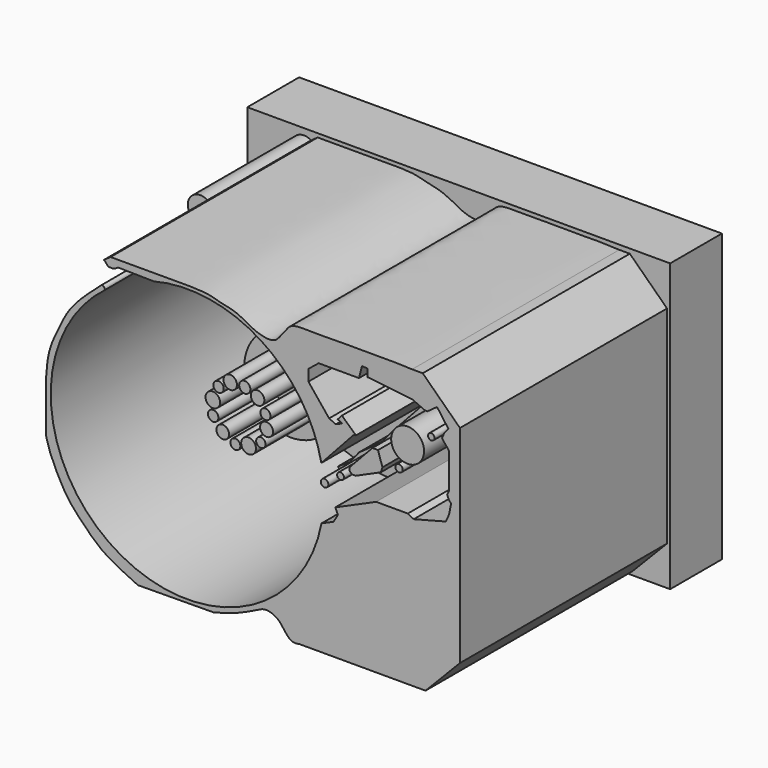
from build123d import *

# Parameters (mm, degrees)
F0_W     = 165.9392981062
F0_H     = 112.5707998872
F1_DEPTH = 25.4
F0_R     = 18.362033197
F2_DEPTH = 25.4
F0_R_2   = 1.3245760179
F0_R_3   = 1.6180887527
F0_R_4   = 1.5016288639
F0_R_5   = 1.5308685242
F0_R_6   = 1.423680284
F0_R_7   = 1.8647629935
F0_R_8   = 2.0434590637
F3_DEPTH = 101.6
F0_R_9   = 2.8584843347
F0_R_10  = 2.033776086
F0_R_11  = 2.6280999476
F0_R_12  = 2.1900875489
F0_R_13  = 2.646289047
F0_R_14  = 1.983205802
F0_R_15  = 2.5672784981
F0_R_16  = 1.8338916461
F0_R_17  = 2.9015877895
F0_R_18  = 1.9588755687
F0_R_19  = 2.4970768298
F0_R_20  = 1.4334147906
F0_R_21  = 6.4546403477
F0_R_22  = 1.275539693
F0_R_23  = 1.4866669549
F0_R_24  = 1.3335540023
F4_DEPTH = 76.2
F0_R_25  = 2.3077206763
F5_DEPTH = 127


# Not quite as in the source:
# - a feature names something its author has since deleted; it is built from what else it names


with BuildPart() as f1:
    # F0 (on Front) → F1 (new body)
    with BuildSketch(Plane.XZ):
        with Locations((-83.9341042461, -56.6721437499)):
            Rectangle(F0_W, F0_H)
        with BuildLine():
            add(Edge.make_bspline(
                [(-164.598762989, -71.9534307718), (-164.6019804727, -70.301781771), (-164.6090784651, -66.6581294606), (-164.5482157868, -58.819482394), (-164.7950691846, -52.0330130517), (-163.7374427264, -41.4198242134), (-160.0827700828, -34.2963401288), (-156.4790843754, -26.1909418494), (-150.7406910055, -19.6763424087), (-145.530215111, -15.0828061332), (-142.7876929211, -12.6653148558)],
                knots=[0, 0, 0, 0, 0.1000210606, 0.2206534006, 0.3367660722, 0.4769540157, 0.6014757189, 0.7294078454, 0.8575200865, 0.9998406243, 0.9998406243, 0.9998406243, 0.9998406243], degree=3))
            add(Edge.make_bspline(
                [(-143.3946741623, -12.5450599833), (-143.1883174895, -12.5826121553), (-142.9822493327, -12.6205904733), (-142.7876929211, -12.6653148558)],
                knots=[0, 0, 0, 0, 0.1891030532, 0.1891030532, 0.1891030532, 0.1891030532], degree=3))
            ThreePointArc((-143.3946741623, -12.5450599833), (-149.5463977213, -6.9914400334), (-141.9263395611, -3.7324354414))
            Line((-141.9263395611, -3.7324354414), (-139.2825245857, -1.8620226765))
            add(Edge.make_bspline(
                [(-139.2825245857, -1.8620226765), (-136.5395607147, -1.8628613769), (-130.4584942921, -1.8647207497), (-117.4190427855, -1.8500489741), (-110.495055532, -1.8905468427), (-106.0578439103, -1.7735924347), (-100.2520493143, -2.2187206408), (-96.5814322262, -3.5750412815), (-91.8177960869, -4.2369226936), (-87.1565766192, -6.2408038722), (-83.7146728479, -8.3917462542), (-80.2039650745, -9.7577587847), (-74.7501088384, -10.6611105909), (-72.0211091883, -6.5408088644), (-70.0817167302, -4.1727022961), (-67.8282888978, -1.5520558306), (-57.6837259787, -2.2476289823), (-49.8219729842, -1.7591343826), (-37.8466777831, -2.1896007905), (-29.9600520641, -1.7316118376), (-23.4707458973, -2.1886006133), (-20.9419615567, -2.1850855555)],
                knots=[0, 0, 0, 0, 0.0604152758, 0.1339388058, 0.1870270437, 0.2294758615, 0.2776594332, 0.3179706024, 0.3620093694, 0.4077635186, 0.4481802316, 0.4879171376, 0.5330108477, 0.5757838582, 0.6112628399, 0.6462449623, 0.7084529789, 0.7682332833, 0.8371419361, 0.8957157052, 0.9554909702, 0.9554909702, 0.9554909702, 0.9554909702], degree=3))
            Line((-20.9419615567, -2.1850855555), (-16.7830623686, -2.1850855555))
            Line((-16.7830623686, -2.1850855555), (-2.1772154141, -16.3455307484))
            Line((-2.1772154141, -16.3455307484), (-2.1772154141, -97.562648356))
            Line((-2.1772154141, -97.562648356), (-15.691463348, -111.5019726032))
            Line((-15.691463348, -111.5019726032), (-65.0405287743, -111.5019726032))
            add(Edge.make_bspline(
                [(-65.0405287743, -111.5019726032), (-66.0427724905, -111.6729488277), (-68.18183021, -112.0378580877), (-70.9494266384, -109.0193142343), (-72.9618898641, -105.9323198849), (-75.8020531619, -104.1920869617), (-78.9146757006, -103.7264425867), (-81.3008741463, -104.8100915248), (-84.589202856, -106.5637239353), (-91.0030309407, -109.3941310665), (-94.7401073295, -110.1532539678), (-97.5532729283, -111.2714741148), (-99.0120321512, -111.5019726032)],
                knots=[0, 0, 0, 0, 0.0797931353, 0.1703000171, 0.2607401056, 0.3444672255, 0.4247989579, 0.4975922546, 0.5885406385, 0.7114831575, 0.8042636185, 0.9015998744, 0.9015998744, 0.9015998744, 0.9015998744], degree=3))
            add(Edge.make_bspline(
                [(-99.0120321512, -111.5019726032), (-100.3435178634, -111.712360609), (-101.6903914662, -111.637814719), (-103.0387594819, -111.5355971431)],
                knots=[0.9015998744, 0.9015998744, 0.9015998744, 0.9015998744, 0.9904437576, 0.9904437576, 0.9904437576, 0.9904437576], degree=3))
            Line((-103.0387594819, -111.5355971431), (-128.5932660103, -111.7489859462))
            add(Edge.make_bspline(
                [(-164.598762989, -71.9534307718), (-164.1152431597, -73.7441624945), (-162.9776573937, -77.9571274534), (-157.8950585147, -88.3556118532), (-152.670446881, -95.1120772869), (-143.6170014595, -103.9455151645), (-138.2315033827, -107.0057358427), (-132.0264786482, -110.2505102754), (-128.5932660103, -111.7489859462)],
                knots=[0, 0, 0, 0, 0.1365777233, 0.3213469317, 0.4888780091, 0.6804373106, 0.8201790113, 1, 1, 1, 1], degree=3))
        make_face(mode=Mode.SUBTRACT)
        with BuildLine():
            Line((-99.0120321512, -111.5019726032), (-103.0387594819, -111.5355971431))
            add(Edge.make_bspline(
                [(-99.0120321512, -111.5019726032), (-100.3435178634, -111.712360609), (-101.6903914662, -111.637814719), (-103.0387594819, -111.5355971431)],
                knots=[0.9015998744, 0.9015998744, 0.9015998744, 0.9015998744, 0.9904437576, 0.9904437576, 0.9904437576, 0.9904437576], degree=3))
        make_face()
    extrude(amount=F1_DEPTH)


with BuildPart() as f2:
    # F0 (on Front) → F2 (new body)
    with BuildSketch(Plane.XZ):
        with BuildLine():
            Line((-70.1977387071, -60.9718747437), (-56.574680724, -46.1265275587))
            ThreePointArc((-56.574680724, -46.1265275587), (-64.9234452171, -26.3904519564), (-80.3334944937, -11.4993495783))
            ThreePointArc((-80.3334944937, -11.4993495783), (-100.6388609352, -3.7830882793), (-122.3391934331, -4.7547694212))
            ThreePointArc((-122.3391934331, -4.7547694212), (-132.366882023, -8.3962929683), (-141.4752351143, -13.9508529117))
            ThreePointArc((-141.4752351143, -13.9508529117), (-137.5275163475, -102.222520945), (-56.5035421887, -66.9721667291))
            Line((-56.5035421887, -66.9721667291), (-63.1717741489, -69.8296055198))
            Line((-63.1717741489, -69.8296055198), (-65.3577074409, -69.8296055198))
            Line((-65.3577074409, -69.8296055198), (-70.4351824656, -72.0765446916))
            Line((-70.4351824656, -72.0765446916), (-73.1969177723, -74.1202300196))
            Line((-73.1969177723, -74.1202300196), (-74.5580455289, -74.1202300196))
            Line((-74.5580455289, -74.1202300196), (-75.835108757, -75.0652573638))
            Line((-75.835108757, -75.0652573638), (-76.5364761779, -74.1174641089))
            Line((-76.5364761779, -74.1174641089), (-79.6039626002, -76.3874053955))
            Line((-79.6039626002, -76.3874053955), (-84.8007247001, -78.5980582443))
            Line((-84.8007247001, -78.5980582443), (-89.1530732694, -81.3880295523))
            Line((-89.1530732694, -81.3880295523), (-90.6585007906, -79.0395662189))
            Line((-90.6585007906, -79.0395662189), (-85.9920158982, -76.0482251644))
            Line((-85.9920158982, -76.0482251644), (-82.402408123, -71.5013891459))
            Line((-82.402408123, -71.5013891459), (-78.8128003478, -68.9886659384))
            Line((-78.8128003478, -68.9886659384), (-73.0694234371, -64.5614787936))
            Line((-73.0694234371, -64.5614787936), (-70.1977387071, -60.9718747437))
        make_face()
        with Locations((-109.1400161386, -56.7288547754)):
            Circle(F0_R, mode=Mode.SUBTRACT)
    extrude(amount=F2_DEPTH)


with BuildPart() as f2b:
    # F0 (on Front) → F2, piece 2 (new body)
    with BuildSketch(Plane.XZ):
        Polygon((-48.49641552, -27.1187333148), (-42.9847687483, -32.1765795624), (-40.6026027368, -32.1765795624), (-35.0471251359, -35.0970716348), (-32.0976511653, -37.8037011545), (-30.0747426595, -42.3621244885), (-27.5550070603, -48.0400983156), (-22.6341634989, -52.5557850373), (-20.3160108814, -53.7547796489), (-7.7129306113, -50.4702657487), (-6.476437673, -47.710724175), (-5.6200611483, -43.5287441048), (-6.476437673, -42.7428771995), (-7.2142304973, -41.0803343724), (-6.476437673, -39.4337661564), (-6.476437673, -25.5898251185), (-9.2489010171, -22.1552284073), (-8.2715748094, -19.9740818615), (-6.7090789214, -18.1127964376), (-11.1667942256, -11.9998203591), (-15.0142415941, -14.8054627821), (-16.0565747822, -14.6709703758), (-17.4124831619, -14.0634161529), (-20.8762927528, -12.5113554267), (-35.0471251359, -10.9489776797), (-38.3834416892, -10.5811385438), (-38.3834416892, -7.5878729292), (-40.6026027368, -7.4437292861), (-41.8101128024, -11.9998203591), (-42.4804815882, -14.5292081691), (-44.9977574558, -14.0634161529), (-50.1625005514, -25.5898251185), align=None)
        with Locations((-11.93417795, -42.617212981)):
            Circle(F0_R_2, mode=Mode.SUBTRACT)
        with Locations((-10.1036969572, -38.558319211)):
            Circle(F0_R_3, mode=Mode.SUBTRACT)
        with Locations((-44.0073870122, -21.6064751148)):
            Circle(F0_R_4, mode=Mode.SUBTRACT)
        with Locations((-35.6508418918, -16.6721362621)):
            Circle(F0_R_5, mode=Mode.SUBTRACT)
        with Locations((-31.5123647451, -15.0008266792)):
            Circle(F0_R_6, mode=Mode.SUBTRACT)
        Polygon((-50.1625005514, -28.9343029733), (-48.49641552, -27.1187333148), (-50.1625005514, -25.5898251185), (-44.9977574558, -14.0634161529), (-42.4804815882, -14.5292081691), (-41.8101128024, -11.9998203591), (-57.6271012125, -11.9998203591), (-61.6406015034, -15.2395842597), (-61.6406015034, -19.6711045673), (-53.5235144198, -29.7267544143), (-50.8820651749, -30.9103326467), (-48.3049005871, -29.7666547161), align=None)
        with Locations((-54.9106858671, -16.7517215014)):
            Circle(F0_R_7, mode=Mode.SUBTRACT)
    extrude(amount=F2_DEPTH)


with BuildPart() as f3:
    # F0 (on Front) → F3 (new body)
    with BuildSketch(Plane.XZ):
        with Locations((-119.3423271179, -60.5702623725)):
            Circle(F0_R_8)
    extrude(amount=F3_DEPTH)


with BuildPart() as f3b:
    # F0 (on Front) → F3, piece 2 (new body)
    with BuildSketch(Plane.XZ):
        with Locations((-119.4925680757, -55.0865530968)):
            Circle(F0_R_9)
    extrude(amount=F3_DEPTH)


with BuildPart() as f3c:
    # F0 (on Front) → F3, piece 3 (new body)
    with BuildSketch(Plane.XZ):
        with Locations((-117.2389909625, -49.9033220112)):
            Circle(F0_R_10)
    extrude(amount=F3_DEPTH)


with BuildPart() as f3d:
    # F0 (on Front) → F3, piece 4 (new body)
    with BuildSketch(Plane.XZ):
        with Locations((-112.656712532, -46.8234308064)):
            Circle(F0_R_11)
    extrude(amount=F3_DEPTH)


with BuildPart() as f3e:
    # F0 (on Front) → F3, piece 5 (new body)
    with BuildSketch(Plane.XZ):
        with Locations((-106.947645545, -46.673193574)):
            Circle(F0_R_12)
    extrude(amount=F3_DEPTH)


with BuildPart() as f3f:
    # F0 (on Front) → F3, piece 6 (new body)
    with BuildSketch(Plane.XZ):
        with Locations((-101.9146516919, -48.7014129758)):
            Circle(F0_R_13)
    extrude(amount=F3_DEPTH)


with BuildPart() as f3g:
    # F0 (on Front) → F3, piece 7 (new body)
    with BuildSketch(Plane.XZ):
        with Locations((-98.8347604871, -53.3588118851)):
            Circle(F0_R_14)
    extrude(amount=F3_DEPTH)


with BuildPart() as f3h:
    # F0 (on Front) → F3, piece 8 (new body)
    with BuildSketch(Plane.XZ):
        with Locations((-98.3840450644, -58.4669224918)):
            Circle(F0_R_15)
    extrude(amount=F3_DEPTH)


with BuildPart() as f3i:
    # F0 (on Front) → F3, piece 9 (new body)
    with BuildSketch(Plane.XZ):
        with Locations((-100.6376221776, -63.7252777815)):
            Circle(F0_R_16)
    extrude(amount=F3_DEPTH)


with BuildPart() as f3j:
    # F0 (on Front) → F3, piece 10 (new body)
    with BuildSketch(Plane.XZ):
        with Locations((-105.4452583194, -66.4295703173)):
            Circle(F0_R_17)
    extrude(amount=F3_DEPTH)


with BuildPart() as f3k:
    # F0 (on Front) → F3, piece 11 (new body)
    with BuildSketch(Plane.XZ):
        with Locations((-110.6284931302, -67.5563588738)):
            Circle(F0_R_18)
    extrude(amount=F3_DEPTH)


with BuildPart() as f3l:
    # F0 (on Front) → F3, piece 12 (new body)
    with BuildSketch(Plane.XZ):
        with Locations((-115.5863627791, -64.9271830916)):
            Circle(F0_R_19)
    extrude(amount=F3_DEPTH)


with BuildPart() as f3m:
    # F0 (on Front) → F3, piece 13 (new body)
    with BuildSketch(Plane.XZ):
        with BuildLine():
            ThreePointArc((-55.5161051505, -56.7288547754), (-55.5835510395, -54.040197908), (-55.7857190454, -51.3583043986))
            Line((-55.7857190454, -51.3583043986), (-56.8401031196, -51.3583043986))
            Line((-56.8401031196, -51.3583043986), (-65.8099651337, -60.935113579))
            Line((-65.8099651337, -60.935113579), (-65.8099651337, -62.2165240347))
            Line((-65.8099651337, -62.2165240347), (-64.861602465, -63.0868034201))
            Line((-64.861602465, -63.0868034201), (-63.3979067206, -63.0868034201))
            Line((-63.3979067206, -63.0868034201), (-55.592952435, -59.59866285))
            ThreePointArc((-55.592952435, -59.59866285), (-55.5353204143, -58.1642731718), (-55.5161051505, -56.7288547754))
        make_face()
        with BuildLine():
            Line((-54.6272667849, -51.3583043986), (-55.7857190454, -51.3583043986))
            ThreePointArc((-55.7857190454, -51.3583043986), (-55.5835510395, -54.040197908), (-55.5161051505, -56.7288547754))
            ThreePointArc((-55.5161051505, -56.7288547754), (-55.5353204143, -58.1642731718), (-55.592952435, -59.59866285))
            Line((-55.592952435, -59.59866285), (-53.5235144198, -58.6738027632))
            Line((-53.5235144198, -58.6738027632), (-52.9269772227, -56.7833116211))
            Line((-52.9269772227, -56.7833116211), (-54.6272667849, -51.3583043986))
        make_face()
    extrude(amount=F3_DEPTH)


with BuildPart() as f3n:
    # F0 (on Front) → F3, piece 14 (new body)
    with BuildSketch(Plane.XZ):
        with Locations((-46.3980771601, -54.993160069)):
            Circle(F0_R_20)
    extrude(amount=F3_DEPTH)


with BuildPart() as f3o:
    # F0 (on Front) → F3, piece 15 (new body)
    with BuildSketch(Plane.XZ):
        with Locations((-43.0253371596, -45.8867549896)):
            Circle(F0_R_21)
    extrude(amount=F3_DEPTH)


with BuildPart() as f3p:
    # F0 (on Front) → F3, piece 16 (new body)
    with BuildSketch(Plane.XZ):
        with Locations((-33.7502919137, -39.9844571948)):
            Circle(F0_R_22)
    extrude(amount=F3_DEPTH)


with BuildPart() as f3q:
    # F0 (on Front) → F3, piece 17 (new body)
    with BuildSketch(Plane.XZ):
        with Locations((-75.6089836359, -69.6034729481)):
            Circle(F0_R_23)
    extrude(amount=F3_DEPTH)


with BuildPart() as f3r:
    # F0 (on Front) → F3, piece 18 (new body)
    with BuildSketch(Plane.XZ):
        with Locations((-69.3526864052, -65.1562288404)):
            Circle(F0_R_24)
    extrude(amount=F3_DEPTH)


with BuildPart() as f3s:
    # F0 (on Front) → F3, piece 19 (new body)
    with BuildSketch(Plane.XZ):
        with Locations((-54.9106858671, -16.7517215014)):
            Circle(F0_R_7)
    extrude(amount=F3_DEPTH)


with BuildPart() as f3t:
    # F0 (on Front) → F3, piece 20 (new body)
    with BuildSketch(Plane.XZ):
        with Locations((-44.0073870122, -21.6064751148)):
            Circle(F0_R_4)
    extrude(amount=F3_DEPTH)


with BuildPart() as f3u:
    # F0 (on Front) → F3, piece 21 (new body)
    with BuildSketch(Plane.XZ):
        with Locations((-35.6508418918, -16.6721362621)):
            Circle(F0_R_5)
    extrude(amount=F3_DEPTH)


with BuildPart() as f3v:
    # F0 (on Front) → F3, piece 22 (new body)
    with BuildSketch(Plane.XZ):
        with Locations((-31.5123647451, -15.0008266792)):
            Circle(F0_R_6)
    extrude(amount=F3_DEPTH)


with BuildPart() as f3w:
    # F0 (on Front) → F3, piece 23 (new body)
    with BuildSketch(Plane.XZ):
        with Locations((-10.1036969572, -38.558319211)):
            Circle(F0_R_3)
    extrude(amount=F3_DEPTH)


with BuildPart() as f3x:
    # F0 (on Front) → F3, piece 24 (new body)
    with BuildSketch(Plane.XZ):
        with Locations((-11.93417795, -42.617212981)):
            Circle(F0_R_2)
    extrude(amount=F3_DEPTH)


with BuildPart() as f4:
    # F0 (on Front) → F4 (new body)
    with BuildSketch(Plane.XZ):
        with Locations((-109.1400161386, -56.7288547754)):
            Circle(F0_R)
        with Locations((-115.5863627791, -64.9271830916)):
            Circle(F0_R_19, mode=Mode.SUBTRACT)
        with Locations((-110.6284931302, -67.5563588738)):
            Circle(F0_R_18, mode=Mode.SUBTRACT)
        with Locations((-105.4452583194, -66.4295703173)):
            Circle(F0_R_17, mode=Mode.SUBTRACT)
        with Locations((-119.3423271179, -60.5702623725)):
            Circle(F0_R_8, mode=Mode.SUBTRACT)
        with Locations((-100.6376221776, -63.7252777815)):
            Circle(F0_R_16, mode=Mode.SUBTRACT)
        with Locations((-98.3840450644, -58.4669224918)):
            Circle(F0_R_15, mode=Mode.SUBTRACT)
        with Locations((-119.4925680757, -55.0865530968)):
            Circle(F0_R_9, mode=Mode.SUBTRACT)
        with Locations((-117.2389909625, -49.9033220112)):
            Circle(F0_R_10, mode=Mode.SUBTRACT)
        with Locations((-112.656712532, -46.8234308064)):
            Circle(F0_R_11, mode=Mode.SUBTRACT)
        with Locations((-106.947645545, -46.673193574)):
            Circle(F0_R_12, mode=Mode.SUBTRACT)
        with Locations((-98.8347604871, -53.3588118851)):
            Circle(F0_R_14, mode=Mode.SUBTRACT)
        with Locations((-101.9146516919, -48.7014129758)):
            Circle(F0_R_13, mode=Mode.SUBTRACT)
    extrude(amount=F4_DEPTH)


with BuildPart() as f4b:
    # F0 (on Front) → F4, piece 2 (new body)
    with BuildSketch(Plane.XZ):
        with BuildLine():
            Line((-43.7732993857, -32.1765795624), (-56.574680724, -46.1265275587))
            ThreePointArc((-56.574680724, -46.1265275587), (-56.115634861, -48.732679453), (-55.7857190454, -51.3583043986))
            Line((-55.7857190454, -51.3583043986), (-54.6272667849, -51.3583043986))
            Line((-54.6272667849, -51.3583043986), (-52.9269772227, -56.7833116211))
            Line((-52.9269772227, -56.7833116211), (-53.5235144198, -58.6738027632))
            Line((-53.5235144198, -58.6738027632), (-55.592952435, -59.59866285))
            ThreePointArc((-55.592952435, -59.59866285), (-55.7081022731, -61.2625519791), (-55.8749422333, -62.9220552019))
            ThreePointArc((-55.8749422333, -62.9220552019), (-56.1505331219, -64.9531188326), (-56.5035421887, -66.9721667291))
            Line((-56.5035421887, -66.9721667291), (-51.7646975374, -64.8691919831))
            Line((-51.7646975374, -64.8691919831), (-50.0711912212, -61.9773715197))
            Line((-50.0711912212, -61.9773715197), (-51.0923712868, -59.6762437001))
            Line((-51.0923712868, -59.6762437001), (-35.0471251359, -52.5557850373))
            Line((-35.0471251359, -52.5557850373), (-22.6341634989, -52.5557850373))
            Line((-22.6341634989, -52.5557850373), (-27.5550070603, -48.0400983156))
            Line((-27.5550070603, -48.0400983156), (-30.0747426595, -42.3621244885))
            Line((-30.0747426595, -42.3621244885), (-32.0976511653, -37.8037011545))
            Line((-32.0976511653, -37.8037011545), (-35.0471251359, -35.0970716348))
            Line((-35.0471251359, -35.0970716348), (-40.6026027368, -32.1765795624))
            Line((-40.6026027368, -32.1765795624), (-42.9847687483, -32.1765795624))
            Line((-42.9847687483, -32.1765795624), (-43.7732993857, -32.1765795624))
        make_face()
        with Locations((-46.3980771601, -54.993160069)):
            Circle(F0_R_20, mode=Mode.SUBTRACT)
        with Locations((-43.0253371596, -45.8867549896)):
            Circle(F0_R_21, mode=Mode.SUBTRACT)
        with Locations((-33.7502919137, -39.9844571948)):
            Circle(F0_R_22, mode=Mode.SUBTRACT)
        with BuildLine():
            ThreePointArc((-55.7857190454, -51.3583043986), (-56.115634861, -48.732679453), (-56.574680724, -46.1265275587))
            Line((-56.574680724, -46.1265275587), (-70.1977387071, -60.9718747437))
            Line((-70.1977387071, -60.9718747437), (-73.0694234371, -64.5614787936))
            Line((-73.0694234371, -64.5614787936), (-78.8128003478, -68.9886659384))
            Line((-78.8128003478, -68.9886659384), (-82.402408123, -71.5013891459))
            Line((-82.402408123, -71.5013891459), (-85.9920158982, -76.0482251644))
            Line((-85.9920158982, -76.0482251644), (-90.6585007906, -79.0395662189))
            Line((-90.6585007906, -79.0395662189), (-89.1530732694, -81.3880295523))
            Line((-89.1530732694, -81.3880295523), (-84.8007247001, -78.5980582443))
            Line((-84.8007247001, -78.5980582443), (-79.6039626002, -76.3874053955))
            Line((-79.6039626002, -76.3874053955), (-76.5364761779, -74.1174641089))
            Line((-76.5364761779, -74.1174641089), (-75.835108757, -73.5984519124))
            Line((-75.835108757, -73.5984519124), (-70.1977387071, -69.0004602075))
            Line((-70.1977387071, -69.0004602075), (-65.0561973453, -66.9652745128))
            Line((-65.0561973453, -66.9652745128), (-63.3225291967, -67.568294704))
            Line((-63.3225291967, -67.568294704), (-61.5888535976, -66.814519465))
            Line((-61.5888535976, -66.814519465), (-61.5888535976, -65.4577389359))
            Line((-61.5888535976, -65.4577389359), (-55.8749422333, -62.9220552019))
            ThreePointArc((-55.8749422333, -62.9220552019), (-55.7081022731, -61.2625519791), (-55.592952435, -59.59866285))
            Line((-55.592952435, -59.59866285), (-63.3979067206, -63.0868034201))
            Line((-63.3979067206, -63.0868034201), (-64.861602465, -63.0868034201))
            Line((-64.861602465, -63.0868034201), (-65.8099651337, -62.2165240347))
            Line((-65.8099651337, -62.2165240347), (-65.8099651337, -60.935113579))
            Line((-65.8099651337, -60.935113579), (-56.8401031196, -51.3583043986))
            Line((-56.8401031196, -51.3583043986), (-55.7857190454, -51.3583043986))
        make_face()
        with Locations((-75.6089836359, -69.6034729481)):
            Circle(F0_R_23, mode=Mode.SUBTRACT)
        with Locations((-69.3526864052, -65.1562288404)):
            Circle(F0_R_24, mode=Mode.SUBTRACT)
        with BuildLine():
            Line((-63.1717741489, -69.8296055198), (-56.5035421887, -66.9721667291))
            ThreePointArc((-56.5035421887, -66.9721667291), (-56.1505331219, -64.9531188326), (-55.8749422333, -62.9220552019))
            Line((-55.8749422333, -62.9220552019), (-61.5888535976, -65.4577389359))
            Line((-61.5888535976, -65.4577389359), (-61.5888535976, -66.814519465))
            Line((-61.5888535976, -66.814519465), (-63.3225291967, -67.568294704))
            Line((-63.3225291967, -67.568294704), (-65.0561973453, -66.9652745128))
            Line((-65.0561973453, -66.9652745128), (-70.1977387071, -69.0004602075))
            Line((-70.1977387071, -69.0004602075), (-75.835108757, -73.5984519124))
            Line((-75.835108757, -73.5984519124), (-76.5364761779, -74.1174641089))
            Line((-76.5364761779, -74.1174641089), (-75.835108757, -75.0652573638))
            Line((-75.835108757, -75.0652573638), (-74.5580455289, -74.1202300196))
            Line((-74.5580455289, -74.1202300196), (-73.1969177723, -74.1202300196))
            Line((-73.1969177723, -74.1202300196), (-70.4351824656, -72.0765446916))
            Line((-70.4351824656, -72.0765446916), (-65.3577074409, -69.8296055198))
            Line((-65.3577074409, -69.8296055198), (-63.1717741489, -69.8296055198))
        make_face()
    extrude(amount=F4_DEPTH)


with BuildPart() as f4c:
    # F0 (on Front) → F4, piece 3 (new body)
    with BuildSketch(Plane.XZ):
        with BuildLine():
            ThreePointArc((-141.4752351143, -13.9508529117), (-132.366882023, -8.3962929683), (-122.3391934331, -4.7547694212))
            Line((-122.3391934331, -4.7547694212), (-136.2758278847, -4.5380867086))
            add(Edge.make_bspline(
                [(-136.2758278847, -4.5380867086), (-136.9283356938, -4.9395970351), (-138.2189497836, -5.7332343937), (-139.6733716983, -5.5215757827), (-140.3905345542, -5.415407347)],
                knots=[0, 0, 0, 0, 0.50551918, 1, 1, 1, 1], degree=3))
            ThreePointArc((-140.3905345542, -5.415407347), (-139.9306193026, -6.5684919249), (-139.7739897547, -7.7999923378))
            ThreePointArc((-139.7739897547, -7.7999923378), (-140.7825393033, -10.7843273785), (-143.3946741623, -12.5450599833))
            Line((-143.3946741623, -12.5450599833), (-142.7784793903, -12.6571932703))
            add(Edge.make_bspline(
                [(-142.7876929211, -12.6653148558), (-142.7846217445, -12.6626076607), (-142.7815505674, -12.6599004655), (-142.7784793903, -12.6571932703)],
                knots=[0.9998406243, 0.9998406243, 0.9998406243, 0.9998406243, 1, 1, 1, 1], degree=3))
            add(Edge.make_bspline(
                [(-142.7876929211, -12.6653148558), (-142.4012909268, -12.7541404589), (-141.6650490455, -13.0033768935), (-141.5503548031, -13.60746187), (-141.4752351143, -13.9508529117)],
                knots=[0.1891030532, 0.1891030532, 0.1891030532, 0.1891030532, 0.5646743146, 1, 1, 1, 1], degree=3))
        make_face()
        with BuildLine():
            ThreePointArc((-139.7739897547, -7.7999923378), (-139.9306193026, -6.5684919249), (-140.3905345542, -5.415407347))
            ThreePointArc((-140.3905345542, -5.415407347), (-141.0596672582, -4.4837884858), (-141.9263395611, -3.7324354414))
            ThreePointArc((-141.9263395611, -3.7324354414), (-149.5463977213, -6.9914400334), (-143.3946741623, -12.5450599833))
            ThreePointArc((-143.3946741623, -12.5450599833), (-140.7825393033, -10.7843273785), (-139.7739897547, -7.7999923378))
        make_face()
        with Locations((-144.6936428547, -7.7999923378)):
            Circle(F0_R_25, mode=Mode.SUBTRACT)
        with Locations((-144.6936428547, -7.7999923378)):
            Circle(F0_R_25)
    extrude(amount=F4_DEPTH)


with BuildPart() as f5:
    # F0 (on Front) → F5 (new body)
    with BuildSketch(Plane.XZ):
        with BuildLine():
            ThreePointArc((-80.3334944937, -11.4993495783), (-64.9234452171, -26.3904519564), (-56.574680724, -46.1265275587))
            Line((-56.574680724, -46.1265275587), (-43.7732993857, -32.1765795624))
            Line((-43.7732993857, -32.1765795624), (-42.9847687483, -32.1765795624))
            Line((-42.9847687483, -32.1765795624), (-48.49641552, -27.1187333148))
            Line((-48.49641552, -27.1187333148), (-50.1625005514, -28.9343029733))
            Line((-50.1625005514, -28.9343029733), (-48.3049005871, -29.7666547161))
            Line((-48.3049005871, -29.7666547161), (-50.8820651749, -30.9103326467))
            Line((-50.8820651749, -30.9103326467), (-53.5235144198, -29.7267544143))
            Line((-53.5235144198, -29.7267544143), (-61.6406015034, -19.6711045673))
            Line((-61.6406015034, -19.6711045673), (-61.6406015034, -15.2395842597))
            Line((-61.6406015034, -15.2395842597), (-57.6271012125, -11.9998203591))
            Line((-57.6271012125, -11.9998203591), (-41.8101128024, -11.9998203591))
            Line((-41.8101128024, -11.9998203591), (-40.6026027368, -7.4437292861))
            Line((-40.6026027368, -7.4437292861), (-38.3834416892, -7.5878729292))
            Line((-38.3834416892, -7.5878729292), (-38.3834416892, -10.5811385438))
            Line((-38.3834416892, -10.5811385438), (-35.0471251359, -10.9489776797))
            Line((-35.0471251359, -10.9489776797), (-20.8762927528, -12.5113554267))
            Line((-20.8762927528, -12.5113554267), (-17.4124831619, -14.0634161529))
            Line((-17.4124831619, -14.0634161529), (-16.0565747822, -14.6709703758))
            Line((-16.0565747822, -14.6709703758), (-15.0142415941, -14.8054627821))
            Line((-15.0142415941, -14.8054627821), (-11.1667942256, -11.9998203591))
            Line((-11.1667942256, -11.9998203591), (-6.7090789214, -18.1127964376))
            Line((-6.7090789214, -18.1127964376), (-8.2715748094, -19.9740818615))
            Line((-8.2715748094, -19.9740818615), (-9.2489010171, -22.1552284073))
            Line((-9.2489010171, -22.1552284073), (-6.476437673, -25.5898251185))
            Line((-6.476437673, -25.5898251185), (-6.476437673, -39.4337661564))
            Line((-6.476437673, -39.4337661564), (-7.2142304973, -41.0803343724))
            Line((-7.2142304973, -41.0803343724), (-6.476437673, -42.7428771995))
            Line((-6.476437673, -42.7428771995), (-5.6200611483, -43.5287441048))
            Line((-5.6200611483, -43.5287441048), (-6.476437673, -47.710724175))
            Line((-6.476437673, -47.710724175), (-7.7129306113, -50.4702657487))
            Line((-7.7129306113, -50.4702657487), (-20.3160108814, -53.7547796489))
            Line((-20.3160108814, -53.7547796489), (-22.6341634989, -52.5557850373))
            Line((-22.6341634989, -52.5557850373), (-35.0471251359, -52.5557850373))
            Line((-35.0471251359, -52.5557850373), (-51.0923712868, -59.6762437001))
            Line((-51.0923712868, -59.6762437001), (-50.0711912212, -61.9773715197))
            Line((-50.0711912212, -61.9773715197), (-51.7646975374, -64.8691919831))
            Line((-51.7646975374, -64.8691919831), (-56.5035421887, -66.9721667291))
            ThreePointArc((-56.5035421887, -66.9721667291), (-137.5275163475, -102.222520945), (-141.4752351143, -13.9508529117))
            add(Edge.make_bspline(
                [(-142.7876929211, -12.6653148558), (-142.4012909268, -12.7541404589), (-141.6650490455, -13.0033768935), (-141.5503548031, -13.60746187), (-141.4752351143, -13.9508529117)],
                knots=[0.1891030532, 0.1891030532, 0.1891030532, 0.1891030532, 0.5646743146, 1, 1, 1, 1], degree=3))
            add(Edge.make_bspline(
                [(-164.598762989, -71.9534307718), (-164.6019804727, -70.301781771), (-164.6090784651, -66.6581294606), (-164.5482157868, -58.819482394), (-164.7950691846, -52.0330130517), (-163.7374427264, -41.4198242134), (-160.0827700828, -34.2963401288), (-156.4790843754, -26.1909418494), (-150.7406910055, -19.6763424087), (-145.530215111, -15.0828061332), (-142.7876929211, -12.6653148558)],
                knots=[0, 0, 0, 0, 0.1000210606, 0.2206534006, 0.3367660722, 0.4769540157, 0.6014757189, 0.7294078454, 0.8575200865, 0.9998406243, 0.9998406243, 0.9998406243, 0.9998406243], degree=3))
            add(Edge.make_bspline(
                [(-164.598762989, -71.9534307718), (-164.1152431597, -73.7441624945), (-162.9776573937, -77.9571274534), (-157.8950585147, -88.3556118532), (-152.670446881, -95.1120772869), (-143.6170014595, -103.9455151645), (-138.2315033827, -107.0057358427), (-132.0264786482, -110.2505102754), (-128.5932660103, -111.7489859462)],
                knots=[0, 0, 0, 0, 0.1365777233, 0.3213469317, 0.4888780091, 0.6804373106, 0.8201790113, 1, 1, 1, 1], degree=3))
            Line((-128.5932660103, -111.7489859462), (-103.0387594819, -111.5355971431))
            Line((-103.0387594819, -111.5355971431), (-99.0120321512, -111.5019726032))
            add(Edge.make_bspline(
                [(-65.0405287743, -111.5019726032), (-66.0427724905, -111.6729488277), (-68.18183021, -112.0378580877), (-70.9494266384, -109.0193142343), (-72.9618898641, -105.9323198849), (-75.8020531619, -104.1920869617), (-78.9146757006, -103.7264425867), (-81.3008741463, -104.8100915248), (-84.589202856, -106.5637239353), (-91.0030309407, -109.3941310665), (-94.7401073295, -110.1532539678), (-97.5532729283, -111.2714741148), (-99.0120321512, -111.5019726032)],
                knots=[0, 0, 0, 0, 0.0797931353, 0.1703000171, 0.2607401056, 0.3444672255, 0.4247989579, 0.4975922546, 0.5885406385, 0.7114831575, 0.8042636185, 0.9015998744, 0.9015998744, 0.9015998744, 0.9015998744], degree=3))
            Line((-65.0405287743, -111.5019726032), (-15.691463348, -111.5019726032))
            Line((-15.691463348, -111.5019726032), (-2.1772154141, -97.562648356))
            Line((-2.1772154141, -97.562648356), (-2.1772154141, -16.3455307484))
            Line((-2.1772154141, -16.3455307484), (-16.7830623686, -2.1850855555))
            Line((-16.7830623686, -2.1850855555), (-20.9419615567, -2.1850855555))
            add(Edge.make_bspline(
                [(-139.2825245857, -1.8620226765), (-136.5395607147, -1.8628613769), (-130.4584942921, -1.8647207497), (-117.4190427855, -1.8500489741), (-110.495055532, -1.8905468427), (-106.0578439103, -1.7735924347), (-100.2520493143, -2.2187206408), (-96.5814322262, -3.5750412815), (-91.8177960869, -4.2369226936), (-87.1565766192, -6.2408038722), (-83.7146728479, -8.3917462542), (-80.2039650745, -9.7577587847), (-74.7501088384, -10.6611105909), (-72.0211091883, -6.5408088644), (-70.0817167302, -4.1727022961), (-67.8282888978, -1.5520558306), (-57.6837259787, -2.2476289823), (-49.8219729842, -1.7591343826), (-37.8466777831, -2.1896007905), (-29.9600520641, -1.7316118376), (-23.4707458973, -2.1886006133), (-20.9419615567, -2.1850855555)],
                knots=[0, 0, 0, 0, 0.0604152758, 0.1339388058, 0.1870270437, 0.2294758615, 0.2776594332, 0.3179706024, 0.3620093694, 0.4077635186, 0.4481802316, 0.4879171376, 0.5330108477, 0.5757838582, 0.6112628399, 0.6462449623, 0.7084529789, 0.7682332833, 0.8371419361, 0.8957157052, 0.9554909702, 0.9554909702, 0.9554909702, 0.9554909702], degree=3))
            Line((-139.2825245857, -1.8620226765), (-141.9263395611, -3.7324354414))
            ThreePointArc((-141.9263395611, -3.7324354414), (-141.0596672582, -4.4837884858), (-140.3905345542, -5.415407347))
            add(Edge.make_bspline(
                [(-136.2758278847, -4.5380867086), (-136.9283356938, -4.9395970351), (-138.2189497836, -5.7332343937), (-139.6733716983, -5.5215757827), (-140.3905345542, -5.415407347)],
                knots=[0, 0, 0, 0, 0.50551918, 1, 1, 1, 1], degree=3))
            Line((-136.2758278847, -4.5380867086), (-122.3391934331, -4.7547694212))
            ThreePointArc((-122.3391934331, -4.7547694212), (-100.6388609352, -3.7830882793), (-80.3334944937, -11.4993495783))
        make_face()
    extrude(amount=F5_DEPTH)


solid = Compound([f1.part, f2.part, f2b.part, f3.part, f3b.part, f3c.part, f3d.part, f3e.part, f3f.part, f3g.part, f3h.part, f3i.part, f3j.part, f3k.part, f3l.part, f3m.part, f3n.part, f3o.part, f3p.part, f3q.part, f3r.part, f3s.part, f3t.part, f3u.part, f3v.part, f3w.part, f3x.part, f4.part, f4b.part, f4c.part, f5.part])
